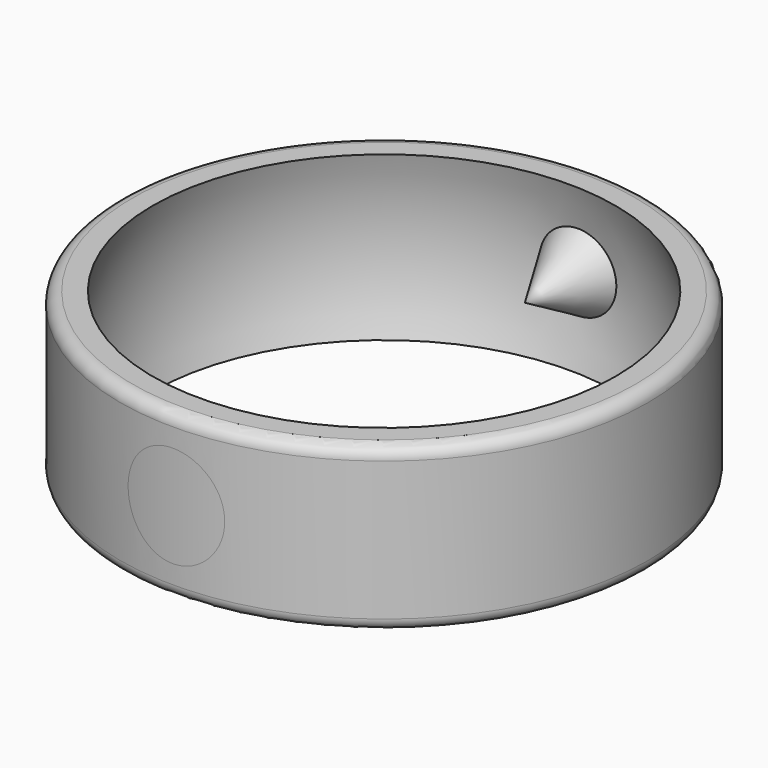
from build123d import *

# Parameters (mm, degrees)
F4_R     = 37.2842712475
F4_R_2   = 32.2842712475
F5_DEPTH = 12.5
F6_R     = 1.5


# Not quite as in the source:
# - a pattern or mirror of a feature is missing from the dataset's text; its kind, count and spacing are read off the source's solid


with BuildPart() as f1:
    # F0 (on Front) → F1 (revolve)
    with BuildSketch(Plane.XZ):
        with BuildLine():
            Line((32.2842712475, 10), (28.2842712475, 10))
            ThreePointArc((28.2842712475, 10), (30, 0), (28.2842712475, -10))
            Line((28.2842712475, -10), (32.2842712475, -10))
            Line((32.2842712475, -10), (32.2842712475, 10))
        make_face()
    revolve(axis=Axis((0, 0, -0.0082536135), (0, 0, -1)))

    # F2 (on Right) → F3 (revolve)
    with BuildSketch(Plane.YZ):
        Polygon((-21.5096189432, 0), (-34.5, 7.5), (-34.5, 0), align=None)
    f3 = revolve(axis=Axis((0, -28.0048094716, 0), (0, -1, 0)))

    # F3_copies: F3 across plane
    add(f3.mirror(Plane.ZX))

    # F4 (on Top) → F5 (cut, symmetric)
    with BuildSketch(Plane.XY):
        Circle(F4_R)
        Circle(F4_R_2, mode=Mode.SUBTRACT)
    extrude(amount=F5_DEPTH, both=True, mode=Mode.SUBTRACT)

    # F6
    f6_edges = [f1.edges().sort_by_distance(p)[0] for p in [
        (-32.284271, 0, 10),
        (-32.284271, 0, -10),
    ]]
    fillet(f6_edges, radius=F6_R)


solid = f1.part
